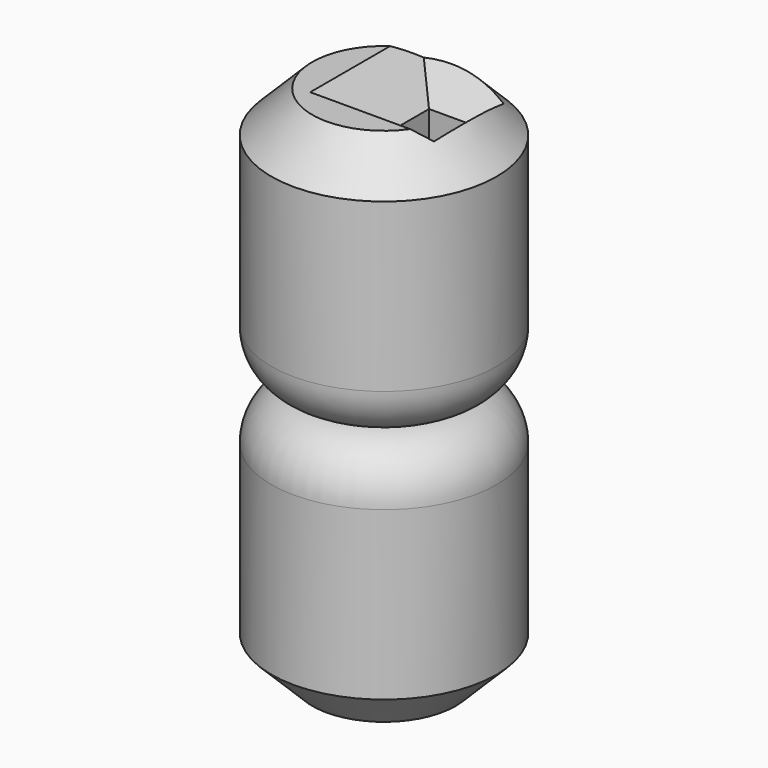
from build123d import *

# Parameters (mm, degrees)
F0_R         = 11
F1_DEPTH     = 25.4
F2_W         = 4.2610359378
F2_H         = 5.4936911911
F1_FACE1_R   = 11
F3_DEPTH     = 25.401
F6_SIZE      = 4
F7_T1_DEPTH  = 5.4936911911
F7_T3_DEPTH  = 4.2610359378
F7_T11_DEPTH = 15.7804231429
F7_S13_R     = 11
F7_T14_DEPTH = 10
F7_T17_DEPTH = 14.5477678897
F7_S19_R     = 11
F7_T20_DEPTH = 9
F7_T26_DEPTH = 15.7804231429
F7_T30_DEPTH = 14.5477678897
F7_T37_DEPTH = 14.5477678897
F7_S39_R     = 11
F7_T40_DEPTH = 9
F7_T43_DEPTH = 15.7804231429
F7_S45_R     = 11
F7_T46_DEPTH = 10
F7_T52_DEPTH = 15.7804231429
F7_S54_R     = 11
F7_T55_DEPTH = 10
F7_T58_DEPTH = 14.5477678897
F7_S60_R     = 11
F7_T61_DEPTH = 9


# Not quite as in the source:
# - a fillet or chamfer that OpenCascade refuses, or shapes differently, is made with other operations: its cross-section is extruded or revolved along the edge and cut away or added


with BuildPart() as f1:
    # F0 (on Top) → F1 (new body)
    with BuildSketch(Plane.XY):
        Circle(F0_R)
    extrude(amount=F1_DEPTH)

    # F2 (on face) + F1_face1 (on face) → F3 (cut, through all)
    with BuildSketch(Plane.XY.offset(25.4)):
        with Locations((2.1305179689, 2.7468455955)):
            Rectangle(F2_W, F2_H)
    with BuildSketch(Plane(origin=(0, 0, 0), x_dir=(1, 0, 0), z_dir=(0, 0, -1))):
        Circle(F1_FACE1_R)
    extrude(amount=-F3_DEPTH, dir=(0, 0, 1), mode=Mode.SUBTRACT)

    # F4: fillet of radius 5.08 on 1 edges, made by hand

    # F4_s1 → F4_t2 (revolve, cut)
    with BuildSketch(Plane.XZ):
        with BuildLine():
            ThreePointArc((11, 5.08), (9.5121024484, 1.4878975516), (5.92, 0))
            Line((5.92, 0), (11, 0))
            Line((11, 0), (11, 5.08))
        make_face()
    revolve(axis=Axis((0, 0, 0), (0, 0, 1)), mode=Mode.SUBTRACT)

    # F5: F1 across face


with BuildPart() as f1_1:
    add(f1.part)
    add(f1.part.mirror(Plane(origin=(-0.5175939516, -0.6620763979, 0), x_dir=(1, 0, 0), z_dir=(0, 0, -1))))

    # F6
    f6_edges = [f1_1.edges().sort_by_distance(p)[0] for p in [
        (-11, 0, -25.4),
    ]]
    chamfer(f6_edges, length=F6_SIZE)

    # F7: chamfer of 4 on 5 edges, made by hand

    # F7_s2 → F7_t1 (cut)
    with BuildSketch(Plane.XZ.offset(-5.4936911911)):
        Polygon((0, 21.4), (-4, 25.4), (0, 25.4), align=None)
        Polygon((4.2610359378, 21.4), (8.2610359378, 25.4), (4.2610359378, 25.4), align=None)
    extrude(amount=F7_T1_DEPTH, mode=Mode.SUBTRACT)

    # F7_s4 → F7_t3 (cut)
    with BuildSketch(Plane.YZ):
        Polygon((0, 21.4), (-4, 25.4), (0, 25.4), align=None)
        Polygon((5.4936911911, 21.4), (9.4936911911, 25.4), (5.4936911911, 25.4), align=None)
    extrude(amount=F7_T3_DEPTH, mode=Mode.SUBTRACT)

    # F7_s5 → F7_t6 (revolve, cut)
    with BuildSketch(Plane.XZ):
        Polygon((7, 25.4), (11, 21.4), (11, 25.4), align=None)
    revolve(axis=Axis((0, 0, 25.4), (0, 0, 1)), mode=Mode.SUBTRACT)


with BuildPart() as f7_tool9:
    # F7_s10 → F7_t11 (new body)
    with BuildSketch(Plane.XZ.offset(-15.7804231429)):
        Polygon((0, 21.4), (-4, 25.4), (0, 25.4), align=None)
    extrude(amount=F7_T11_DEPTH)

    split(bisect_by=Plane.XZ.offset(-5.4936911911), keep=Keep.BOTTOM)

    # F7_s13 → F7_t14 (intersect, symmetric)
    with BuildSketch(Plane.XY.offset(23.4)):
        Circle(F7_S13_R)
    extrude(amount=F7_T14_DEPTH, both=True, mode=Mode.INTERSECT)


with BuildPart() as f7_tool15:
    # F7_s16 → F7_t17 (new body)
    with BuildSketch(Plane.YZ.offset(4.2610359378)):
        Polygon((5.4936911911, 21.4), (9.4936911911, 25.4), (5.4936911911, 25.4), align=None)
    extrude(amount=-F7_T17_DEPTH)

    split(bisect_by=Plane.YZ, keep=Keep.BOTTOM)

    # F7_s19 → F7_t20 (intersect, symmetric)
    with BuildSketch(Plane.XY.offset(23.4)):
        Circle(F7_S19_R)
    extrude(amount=F7_T20_DEPTH, both=True, mode=Mode.INTERSECT)


with BuildPart() as f7_tool9_1:
    add(f7_tool9.part)

    # F7_t21: intersect F7_tool15
    add(f7_tool15.part, mode=Mode.INTERSECT)


with BuildPart() as f1_2:
    add(f1_1.part)

    # F7_t7: cut F7_tool9
    add(f7_tool9_1.part, mode=Mode.SUBTRACT)


with BuildPart() as f7_tool24:
    # F7_s25 → F7_t26 (new body)
    with BuildSketch(Plane.XZ.offset(-5.4936911911)):
        Polygon((0, 21.4), (-4, 25.4), (0, 25.4), align=None)
    extrude(amount=F7_T26_DEPTH)

    split(bisect_by=Plane.XZ, keep=Keep.TOP)


with BuildPart() as f7_tool28:
    # F7_s29 → F7_t30 (new body)
    with BuildSketch(Plane.YZ.offset(-10.2867319519)):
        Polygon((0, 21.4), (-4, 25.4), (0, 25.4), align=None)
    extrude(amount=F7_T30_DEPTH)

    split(bisect_by=Plane.YZ, keep=Keep.BOTTOM)


with BuildPart() as f7_tool24_1:
    add(f7_tool24.part)

    # F7_t32: intersect F7_tool28
    add(f7_tool28.part, mode=Mode.INTERSECT)


with BuildPart() as f1_3:
    add(f1_2.part)

    # F7_t22: cut F7_tool24
    add(f7_tool24_1.part, mode=Mode.SUBTRACT)


with BuildPart() as f7_tool35:
    # F7_s36 → F7_t37 (new body)
    with BuildSketch(Plane.YZ):
        Polygon((0, 21.4), (-4, 25.4), (0, 25.4), align=None)
    extrude(amount=F7_T37_DEPTH)

    split(bisect_by=Plane.YZ.offset(4.2610359378), keep=Keep.TOP)

    # F7_s39 → F7_t40 (intersect, symmetric)
    with BuildSketch(Plane.XY.offset(23.4)):
        Circle(F7_S39_R)
    extrude(amount=F7_T40_DEPTH, both=True, mode=Mode.INTERSECT)


with BuildPart() as f7_tool41:
    # F7_s42 → F7_t43 (new body)
    with BuildSketch(Plane.XZ.offset(10.2867319519)):
        Polygon((4.2610359378, 21.4), (8.2610359378, 25.4), (4.2610359378, 25.4), align=None)
    extrude(amount=-F7_T43_DEPTH)

    split(bisect_by=Plane.XZ, keep=Keep.TOP)

    # F7_s45 → F7_t46 (intersect, symmetric)
    with BuildSketch(Plane.XY.offset(23.4)):
        Circle(F7_S45_R)
    extrude(amount=F7_T46_DEPTH, both=True, mode=Mode.INTERSECT)


with BuildPart() as f7_tool35_1:
    add(f7_tool35.part)

    # F7_t47: intersect F7_tool41
    add(f7_tool41.part, mode=Mode.INTERSECT)


with BuildPart() as f1_4:
    add(f1_3.part)

    # F7_t33: cut F7_tool35
    add(f7_tool35_1.part, mode=Mode.SUBTRACT)


with BuildPart() as f7_tool50:
    # F7_s51 → F7_t52 (new body)
    with BuildSketch(Plane.XZ):
        Polygon((4.2610359378, 21.4), (8.2610359378, 25.4), (4.2610359378, 25.4), align=None)
    extrude(amount=-F7_T52_DEPTH)

    split(bisect_by=Plane.XZ.offset(-5.4936911911), keep=Keep.BOTTOM)

    # F7_s54 → F7_t55 (intersect, symmetric)
    with BuildSketch(Plane.XY.offset(23.4)):
        Circle(F7_S54_R)
    extrude(amount=F7_T55_DEPTH, both=True, mode=Mode.INTERSECT)


with BuildPart() as f7_tool56:
    # F7_s57 → F7_t58 (new body)
    with BuildSketch(Plane.YZ.offset(14.5477678897)):
        Polygon((5.4936911911, 21.4), (9.4936911911, 25.4), (5.4936911911, 25.4), align=None)
    extrude(amount=-F7_T58_DEPTH)

    split(bisect_by=Plane.YZ.offset(4.2610359378), keep=Keep.TOP)

    # F7_s60 → F7_t61 (intersect, symmetric)
    with BuildSketch(Plane.XY.offset(23.4)):
        Circle(F7_S60_R)
    extrude(amount=F7_T61_DEPTH, both=True, mode=Mode.INTERSECT)


with BuildPart() as f7_tool50_1:
    add(f7_tool50.part)

    # F7_t62: intersect F7_tool56
    add(f7_tool56.part, mode=Mode.INTERSECT)


with BuildPart() as f1_5:
    add(f1_4.part)

    # F7_t48: cut F7_tool50
    add(f7_tool50_1.part, mode=Mode.SUBTRACT)


solid = f1_5.part
